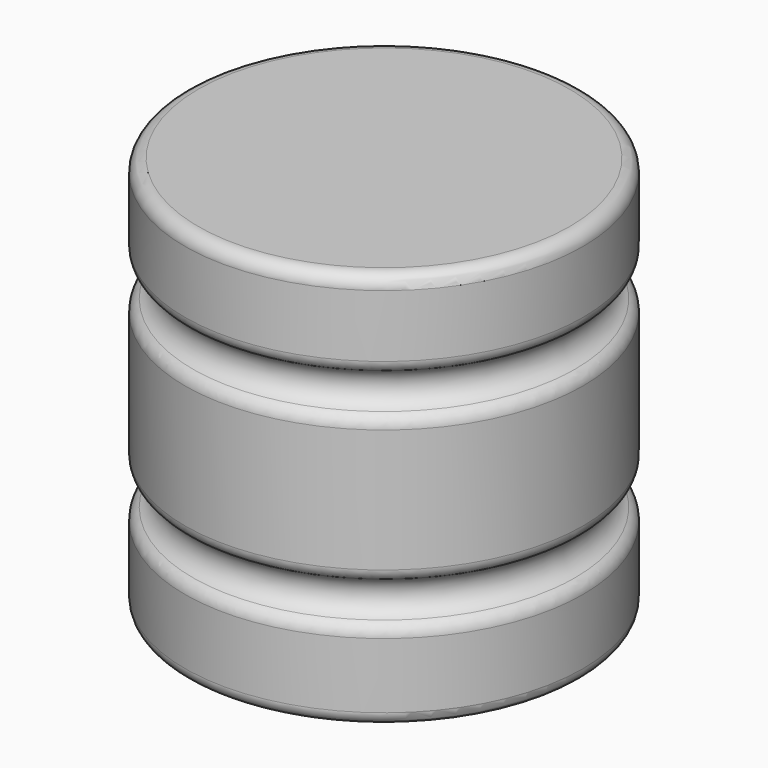
from build123d import *

# Parameters (mm, degrees)
F2_R = 2.54


with BuildPart() as f1:
    # F0 (on Front) → F1 (revolve)
    with BuildSketch(Plane.XZ):
        with BuildLine():
            Line((-38.1, 0), (0, 0))
            Line((0, 0), (0, 17.0421574396))
            ThreePointArc((0, 17.0421574396), (-3.7719, 20.8140574396), (0, 24.5859574396))
            Line((0, 24.5859574396), (0, 52.1778140348))
            ThreePointArc((0, 52.1778140348), (-3.7719, 55.9497140348), (0, 59.7216140348))
            Line((0, 59.7216140348), (0, 76.2))
            Line((0, 76.2), (-38.1, 76.2))
            Line((-38.1, 76.2), (-38.1, 0))
        make_face()
    revolve(axis=Axis((-38.1, 0, 38.1), (0, 0, 1)))

    # F2
    f2_edges = [f1.edges().sort_by_distance(p)[0] for p in [
        (-76.2, 0, 76.2),
        (-76.2, 0, 59.721614),
        (-76.2, 0, 24.585957),
        (-76.2, 0, 0),
        (-76.2, 0, 17.042157),
        (-76.2, 0, 52.177814),
    ]]
    fillet(f2_edges, radius=F2_R)


solid = f1.part
